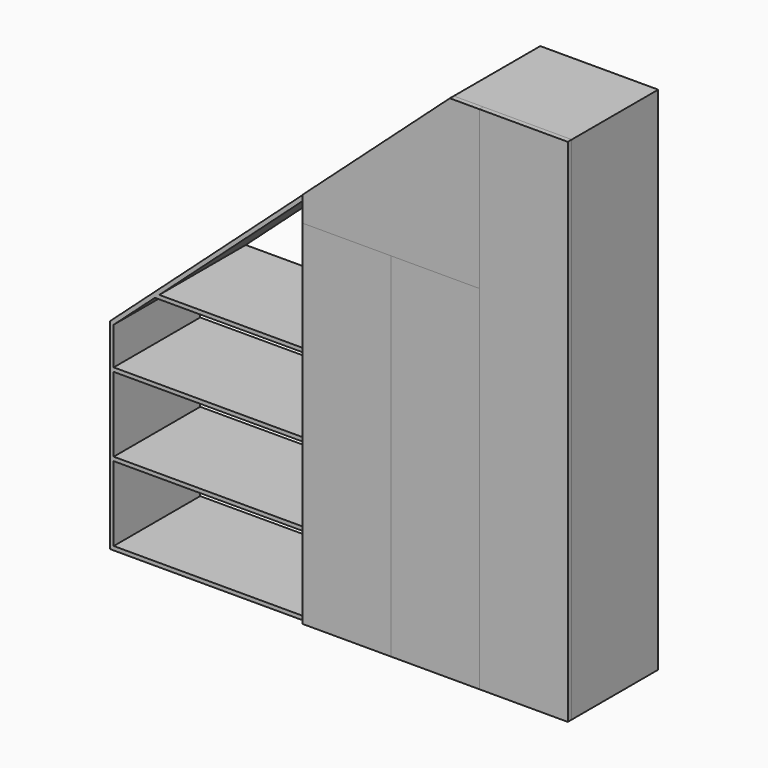
from build123d import *

# Parameters (mm, degrees)
F0_W     = 410
F0_H     = 478
F0_H_2   = 325
F0_H_3   = 330
F0_H_4   = 335
F0_H_5   = 310
F0_W_2   = 960
F0_H_6   = 380
F0_W_3   = 450
F0_H_7   = 20
F1_DEPTH = 550
F2_DEPTH = 25
F0_H_8   = 54.7284266949
F0_H_9   = 960.2715733051
F0_H_10  = 10
F0_H_11  = 250
F0_H_12  = 230
F3_DEPTH = 25
F4_DEPTH = 25
F5_DEPTH = 25


# Not quite as in the source:
# - a feature names something its author has since deleted; it is built from what else it names


with BuildPart() as f1:
    # F0 (on Front) → F1 (new body)
    with BuildSketch(Plane.XZ):
        Polygon((650, 1299), (500, 1299), (200, 1028.4857142857), (200, 1001.5555181998), (507.6855786757, 1279), (650, 1279), align=None)
        Polygon((1100, 1299), (650, 1299), (650, 1279), (650, 516), (650, 496), (650, 441.2715733051), (650, 431.2715733051), (650, -529), (650, -549), (650, -799), (650, -1049), (650, -1279), (650, -1299), (1100, -1299), (1100, -456), (1100, -436), align=None)
        with Locations((875, -1040)):
            Rectangle(F0_W, F0_H, mode=Mode.SUBTRACT)
        with Locations((875, -618.5)):
            Rectangle(F0_W, F0_H_2, mode=Mode.SUBTRACT)
        with Locations((875, -271)):
            Rectangle(F0_W, F0_H_3, mode=Mode.SUBTRACT)
        with Locations((875, 79)):
            Rectangle(F0_W, F0_H_3, mode=Mode.SUBTRACT)
        with Locations((875, 431.5)):
            Rectangle(F0_W, F0_H_4, mode=Mode.SUBTRACT)
        with Locations((875, 784)):
            Rectangle(F0_W, F0_H_3, mode=Mode.SUBTRACT)
        with Locations((875, 1124)):
            Rectangle(F0_W, F0_H_5, mode=Mode.SUBTRACT)
        Polygon((200, 1001.5555181998), (200, 1028.4857142857), (-250, 622.7142857143), (-250, 595.7840896284), align=None)
        Polygon((-250, 595.7840896284), (-250, 622.7142857143), (-1250, -279), (-1250, -479), (-1247.8080965606, -479), (-1230, -462.9421849299), (-1230, -287.8959103716), (-1020.5146748097, -99), (-998.3347001582, -79), (-270, 577.7498039141), align=None)
        Polygon((-250, 516), (-250, 595.7840896284), (-270, 577.7498039141), (-270, -79), (-998.3347001582, -79), (-1020.5146748097, -99), (-270, -99), (-270, -479), (-1230, -479), (-1230, -462.9421849299), (-1247.8080965606, -479), (-1250, -480.9764706442), (-1250, -1299), (-250, -1299), (-250, -1279), (-250, -1049), (-250, -899), (-250, -879), (-250, -799), (-250, -549), (-250, -529), (-250, 431.2715733051), (-250, 441.2715733051), (-250, 496), align=None)
        with Locations((-750, -1089)):
            Rectangle(F0_W_2, F0_H_6, mode=Mode.SUBTRACT)
        with Locations((-750, -689)):
            Rectangle(F0_W_2, F0_H_6, mode=Mode.SUBTRACT)
        Polygon((-1247.8080965606, -479), (-1250, -479), (-1250, -480.9764706442), align=None)
        with Locations((425, -1289)):
            Rectangle(F0_W_3, F0_H_7)
        with Locations((-25, -1289)):
            Rectangle(F0_W_3, F0_H_7)
        with Locations((-25, -539)):
            Rectangle(F0_W_3, F0_H_7)
        with Locations((425, -539)):
            Rectangle(F0_W_3, F0_H_7)
        with Locations((425, 506)):
            Rectangle(F0_W_3, F0_H_7)
        with Locations((-25, 506)):
            Rectangle(F0_W_3, F0_H_7)
    extrude(amount=-F1_DEPTH)


with BuildPart() as f2:
    # F0 (on Front) → F2 (new body)
    with BuildSketch(Plane.XZ):
        Polygon((200, 516), (200, 1001.5555181998), (-250, 595.7840896284), (-250, 516), align=None)
        with Locations((-25, 506)):
            Rectangle(F0_W_3, F0_H_7)
        Polygon((650, 516), (650, 1279), (507.6855786757, 1279), (200, 1001.5555181998), (200, 516), align=None)
        with Locations((425, 506)):
            Rectangle(F0_W_3, F0_H_7)
        Polygon((200, 1001.5555181998), (200, 1028.4857142857), (-250, 622.7142857143), (-250, 595.7840896284), align=None)
        Polygon((650, 1299), (500, 1299), (200, 1028.4857142857), (200, 1001.5555181998), (507.6855786757, 1279), (650, 1279), align=None)
    extrude(amount=F2_DEPTH)


with BuildPart() as f3:
    # F0 (on Front) → F3 (new body)
    with BuildSketch(Plane.XZ):
        with Locations((-25, 468.6357866526)):
            Rectangle(F0_W_3, F0_H_8)
        with Locations((-25, -48.8642133474)):
            Rectangle(F0_W_3, F0_H_9)
        with Locations((-25, 436.2715733051)):
            Rectangle(F0_W_3, F0_H_10)
        with Locations((-25, -674)):
            Rectangle(F0_W_3, F0_H_11)
        Polygon((-250, -1049), (200, -1049), (200, -799), (-250, -799), (-250, -879), (-250, -899), align=None)
        with Locations((-25, -1164)):
            Rectangle(F0_W_3, F0_H_12)
        with Locations((-25, -539)):
            Rectangle(F0_W_3, F0_H_7)
        with Locations((-25, -1289)):
            Rectangle(F0_W_3, F0_H_7)
    extrude(amount=F3_DEPTH)


with BuildPart() as f4:
    # F0 (on Front) → F4 (new body)
    with BuildSketch(Plane.XZ):
        with Locations((425, -1164)):
            Rectangle(F0_W_3, F0_H_12)
        with Locations((425, -924)):
            Rectangle(F0_W_3, F0_H_11)
        with Locations((425, -1289)):
            Rectangle(F0_W_3, F0_H_7)
        with Locations((425, -674)):
            Rectangle(F0_W_3, F0_H_11)
        with Locations((425, -539)):
            Rectangle(F0_W_3, F0_H_7)
        with Locations((425, -48.8642133474)):
            Rectangle(F0_W_3, F0_H_9)
        with Locations((425, 468.6357866526)):
            Rectangle(F0_W_3, F0_H_8)
        with Locations((425, 436.2715733051)):
            Rectangle(F0_W_3, F0_H_10)
    extrude(amount=F4_DEPTH)


with BuildPart() as f5:
    # F0 (on Front) → F5 (new body)
    with BuildSketch(Plane.XZ):
        Polygon((1100, 1299), (650, 1299), (650, 1279), (650, 516), (650, 496), (650, 441.2715733051), (650, 431.2715733051), (650, -529), (650, -549), (650, -799), (650, -1049), (650, -1279), (650, -1299), (1100, -1299), (1100, -456), (1100, -436), align=None)
        with Locations((875, -1040)):
            Rectangle(F0_W, F0_H, mode=Mode.SUBTRACT)
        with Locations((875, -618.5)):
            Rectangle(F0_W, F0_H_2, mode=Mode.SUBTRACT)
        with Locations((875, -271)):
            Rectangle(F0_W, F0_H_3, mode=Mode.SUBTRACT)
        with Locations((875, 79)):
            Rectangle(F0_W, F0_H_3, mode=Mode.SUBTRACT)
        with Locations((875, 431.5)):
            Rectangle(F0_W, F0_H_4, mode=Mode.SUBTRACT)
        with Locations((875, 784)):
            Rectangle(F0_W, F0_H_3, mode=Mode.SUBTRACT)
        with Locations((875, 1124)):
            Rectangle(F0_W, F0_H_5, mode=Mode.SUBTRACT)
        with Locations((875, -1040)):
            Rectangle(F0_W, F0_H)
        with Locations((875, 431.5)):
            Rectangle(F0_W, F0_H_4)
        with Locations((875, 784)):
            Rectangle(F0_W, F0_H_3)
        with Locations((875, 79)):
            Rectangle(F0_W, F0_H_3)
        with Locations((875, -271)):
            Rectangle(F0_W, F0_H_3)
        with Locations((875, -618.5)):
            Rectangle(F0_W, F0_H_2)
        with Locations((875, 1124)):
            Rectangle(F0_W, F0_H_5)
    extrude(amount=F5_DEPTH)


solid = Compound([f1.part, f2.part, f3.part, f4.part, f5.part])
